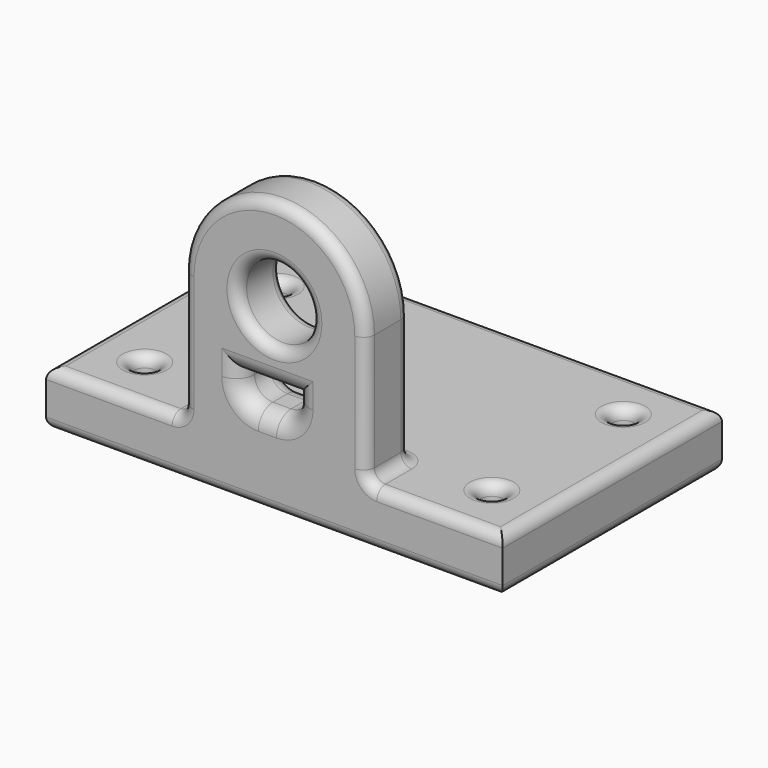
from build123d import *

# Parameters (mm, degrees)
F0_W     = 125
F0_H     = 75
F1_DEPTH = 15
F2_W     = 50
F2_H     = 15
F3_DEPTH = 15
F4_R     = 3
F5_DEPTH = 15
F6_R     = 3
F7_W     = 14.9692930281
F7_H     = 6.8361088634
F8_DEPTH = 25
F9_R     = 5
F10_R    = 5


with BuildPart() as f1:
    # F0 (on Top) → F1 (new body)
    with BuildSketch(Plane.XY):
        Rectangle(F0_W, F0_H)
    extrude(amount=F1_DEPTH)

    # F2 (on face) → F3 (join)
    with BuildSketch(Plane.XZ.offset(37.5)):
        with BuildLine():
            Line((10, 50), (25, 50))
            ThreePointArc((25, 50), (0, 75), (-25, 50))
            Line((-25, 50), (-10, 50))
            ThreePointArc((-10, 50), (0, 60), (10, 50))
        make_face()
        with BuildLine():
            ThreePointArc((-25, 50), (0, 25), (25, 50))
            Line((25, 50), (10, 50))
            ThreePointArc((10, 50), (0, 40), (-10, 50))
            Line((-10, 50), (-25, 50))
        make_face()
        with BuildLine():
            Line((25, 15), (25, 50))
            ThreePointArc((25, 50), (0, 25), (-25, 50))
            Line((-25, 50), (-25, 15))
            Line((-25, 15), (25, 15))
        make_face()
        with Locations((0, 7.5)):
            Rectangle(F2_W, F2_H)
    extrude(amount=-F3_DEPTH)

    # F4 (on face) → F5 (cut, through all)
    with BuildSketch(Plane.XY.offset(15)):
        with Locations((-47.5, -22.5)):
            Circle(F4_R)
        with Locations((47.5, 22.5)):
            Circle(F4_R)
        with Locations((47.5, -22.5)):
            Circle(F4_R)
        with Locations((-47.5, 22.5)):
            Circle(F4_R)
    extrude(amount=-F5_DEPTH, mode=Mode.SUBTRACT)

    # F6
    f6_edges = [f1.edges().sort_by_distance(p)[0] for p in [
        (25, -30, 15),
        (43.75, -37.5, 15),
        (62.5, 0, 15),
        (0, -22.5, 15),
        (0, 37.5, 15),
        (-25, -30, 15),
        (-62.5, 0, 15),
        (-43.75, -37.5, 15),
        (-50.5, -22.5, 15),
        (44.5, -22.5, 15),
        (-50.5, 22.5, 15),
        (44.5, 22.5, 15),
        (62.5, 0, 0),
        (0, -37.5, 0),
        (0, 37.5, 0),
        (-62.5, 0, 0),
        (-50.5, -22.5, 0),
        (44.5, -22.5, 0),
        (-50.5, 22.5, 0),
        (44.5, 22.5, 0),
        (25, -22.5, 32.5),
        (-25, -22.5, 32.5),
        (0, -22.5, 75),
        (-10, -22.5, 50),
        (-10, -37.5, 50),
        (-25, -37.5, 32.5),
        (0, -37.5, 75),
        (25, -37.5, 32.5),
    ]]
    fillet(f6_edges, radius=F6_R)

    # F7 (on face) → F8 (cut)
    with BuildSketch(Plane(origin=(0, -22.5, 0), x_dir=(-1, 0, 0), z_dir=(0, 1, 0))):
        with Locations((1.9257348031, 26.8415547907)):
            Rectangle(F7_W, F7_H)
    extrude(amount=-F8_DEPTH, mode=Mode.SUBTRACT)

    # F9
    f9_edges = [f1.edges().sort_by_distance(p)[0] for p in [
        (-1.925735, -37.5, 30.259609),
        (5.558912, -37.5, 26.841555),
        (-1.925735, -37.5, 23.4235),
        (-9.410381, -37.5, 26.841555),
        (-9.410381, -30, 23.4235),
        (5.558912, -30, 23.4235),
    ]]
    fillet(f9_edges, radius=F9_R)

    # F10
    f10_edges = [f1.edges().sort_by_distance(p)[0] for p in [
        (4.094446, -22.5, 24.887966),
        (-1.925735, -22.5, 30.259609),
        (-9.410381, -22.5, 29.341555),
        (5.558912, -22.5, 29.341555),
        (-7.945915, -22.5, 24.887966),
        (-1.925735, -22.5, 23.4235),
    ]]
    fillet(f10_edges, radius=F10_R)


solid = f1.part
